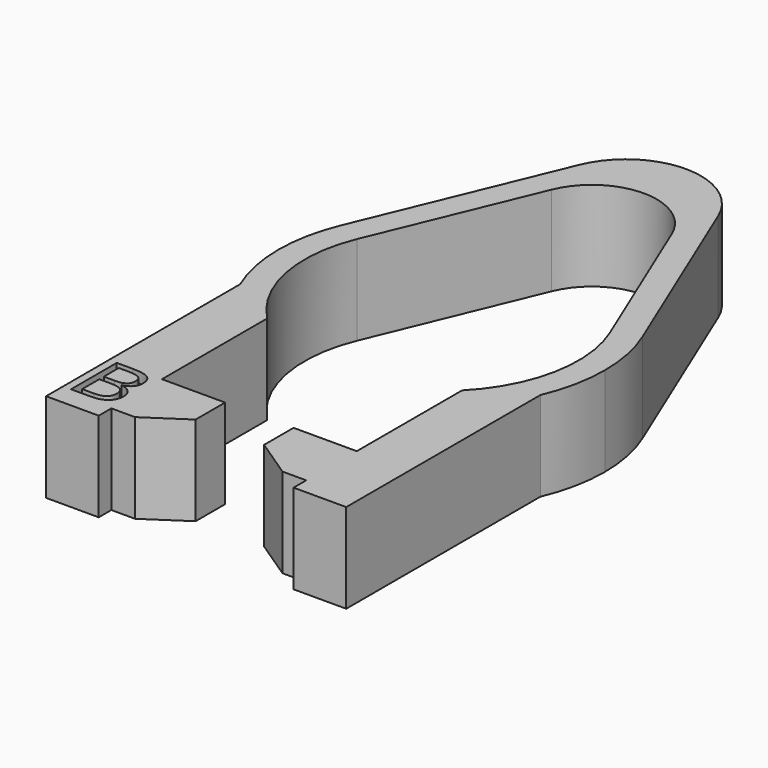
from build123d import *

# Parameters (mm, degrees)
F0_TEXT_SIZE = 7.602755999
F1_DEPTH     = 8.5
F2_DEPTH     = 1


# Not quite as in the source:
# - Text() gives the source's letters only with a copy of the font that has no kerning and outlines rounded to 1/6400 em; it was checked with that copy


with BuildPart() as f1:
    # F0 (on Top) → F1 (new body)
    with BuildSketch(Plane.XY):
        with BuildLine():
            ThreePointArc((-9.25, -9.1344129532), (-12.758649851, -2.493361983), (-12.0083127685, 4.9800024553))
            Line((-12.0083127685, 4.9800024553), (-5.6989333404, 20.1938506868))
            ThreePointArc((-5.6989333404, 20.1938506868), (0, 24), (5.6989333404, 20.1938506868))
            Line((5.6989333404, 20.1938506868), (12.0083127685, 4.9800024553))
            ThreePointArc((12.0083127685, 4.9800024553), (12.758649851, -2.493361983), (9.25, -9.1344129532))
            Line((9.25, -9.1344129532), (9.25, -12.4373429638))
            Line((9.25, -12.4373429638), (9.25, -21.6344129532))
            Line((9.25, -21.6344129532), (3.25, -21.6344129532))
            Line((3.25, -21.6344129532), (3.25, -22.6344129532))
            Line((3.25, -22.6344129532), (3.25, -25.1344129532))
            Line((3.25, -25.1344129532), (7, -27.6344129532))
            Line((7, -27.6344129532), (9.25, -27.6344129532))
            Line((9.25, -27.6344129532), (9.25, -29.1344129532))
            Line((9.25, -29.1344129532), (14.25, -29.1344129532))
            Line((14.25, -29.1344129532), (14.25, -22.6230966869))
            Line((14.25, -22.6230966869), (14.25, -6.0981554588))
            ThreePointArc((14.25, -6.0981554588), (15.1842846391, -3.1124748995), (15.5, 0))
            ThreePointArc((15.5, 0), (15.2015271786, 3.0271391507), (14.3176036855, 5.9376952352))
            Line((14.3176036855, 5.9376952352), (6.5742743873, 24.6092362465))
            ThreePointArc((6.5742743873, 24.6092362465), (0, 29), (-6.5742743873, 24.6092362465))
            Line((-6.5742743873, 24.6092362465), (-14.3176036855, 5.9376952352))
            ThreePointArc((-14.3176036855, 5.9376952352), (-15.2015271786, 3.0271391507), (-15.5, 0))
            ThreePointArc((-15.5, 0), (-15.1842846391, -3.1124748995), (-14.25, -6.0981554588))
            Line((-14.25, -6.0981554588), (-14.25, -22.6344129532))
            Line((-14.25, -22.6344129532), (-14.25, -29.1344129532))
            Line((-14.25, -29.1344129532), (-9.25, -29.1344129532))
            Line((-9.25, -29.1344129532), (-9.25, -27.6344129532))
            Line((-9.25, -27.6344129532), (-7, -27.6344129532))
            Line((-7, -27.6344129532), (-3.25, -25.1344129532))
            Line((-3.25, -25.1344129532), (-3.25, -22.6344129532))
            Line((-3.25, -22.6344129532), (-3.25, -21.6344129532))
            Line((-3.25, -21.6344129532), (-9.25, -21.6344129532))
            Line((-9.25, -21.6344129532), (-9.25, -12.4373429638))
            Line((-9.25, -12.4373429638), (-9.25, -9.1344129532))
        make_face()
        with BuildLine():
            Line((-13.5039795676, -27.1083972725), (-13.5039795676, -21.6807422476))
            Line((-13.5039795676, -21.6807422476), (-11.9703611309, -21.6807422476))
            add(Edge.make_bspline(
                [(-11.9703611309, -21.6807422476), (-10.8905321929, -21.6807422476), (-10.4076383939, -22.0038593776)],
                knots=[0, 0, 0, 1, 1, 1], degree=2))
            add(Edge.make_bspline(
                [(-10.4076383939, -22.0038593776), (-9.9247445949, -22.3269765075), (-9.9247445949, -23.0242917843)],
                knots=[0, 0, 0, 1, 1, 1], degree=2))
            add(Edge.make_bspline(
                [(-9.9247445949, -23.0242917843), (-9.9247445949, -23.5077795486), (-10.1938108814, -23.8213932336)],
                knots=[0, 0, 0, 1, 1, 1], degree=2))
            add(Edge.make_bspline(
                [(-10.1938108814, -23.8213932336), (-10.462877168, -24.1350069185), (-10.9796269898, -24.2276655073)],
                knots=[0, 0, 0, 1, 1, 1], degree=2))
            Line((-10.9796269898, -24.2276655073), (-10.9796269898, -24.2644913566))
            add(Edge.make_bspline(
                [(-10.9796269898, -24.2644913566), (-9.7429912093, -24.4759430079), (-9.7429912093, -25.5640874602)],
                knots=[0, 0, 0, 1, 1, 1], degree=2))
            add(Edge.make_bspline(
                [(-9.7429912093, -25.5640874602), (-9.7429912093, -26.2911010026), (-10.234794488, -26.6997491376)],
                knots=[0, 0, 0, 1, 1, 1], degree=2))
            add(Edge.make_bspline(
                [(-10.234794488, -26.6997491376), (-10.7265977667, -27.1083972725), (-11.6104181516, -27.1083972725)],
                knots=[0, 0, 0, 1, 1, 1], degree=2))
            Line((-11.6104181516, -27.1083972725), (-13.5039795676, -27.1083972725))
        make_face(mode=Mode.SUBTRACT)
        with Locations((-14.25, -27.1083972725)):
            Text('B', F0_TEXT_SIZE, font='Open Sans', text_align=(TextAlign.LEFT, TextAlign.BOTTOM))
        with BuildLine():
            Line((-11.7921715372, -24.538903331), (-12.8731884058, -24.538903331))
            Line((-12.8731884058, -24.538903331), (-12.8731884058, -26.5702646995))
            Line((-12.8731884058, -26.5702646995), (-11.7399025897, -26.5702646995))
            add(Edge.make_bspline(
                [(-11.7399025897, -26.5702646995), (-11.0829769541, -26.5702646995), (-10.7509503445, -26.3160475458)],
                knots=[0, 0, 0, 1, 1, 1], degree=2))
            add(Edge.make_bspline(
                [(-10.7509503445, -26.3160475458), (-10.4189237349, -26.061830392), (-10.4189237349, -25.5189460965)],
                knots=[0, 0, 0, 1, 1, 1], degree=2))
            add(Edge.make_bspline(
                [(-10.4189237349, -25.5189460965), (-10.4189237349, -25.0140755809), (-10.7586718936, -24.776489456)],
                knots=[0, 0, 0, 1, 1, 1], degree=2))
            add(Edge.make_bspline(
                [(-10.7586718936, -24.776489456), (-11.0984200523, -24.538903331), (-11.7921715372, -24.538903331)],
                knots=[0, 0, 0, 1, 1, 1], degree=2))
        make_face()
        with BuildLine():
            Line((-12.8731884058, -22.227190335), (-12.8731884058, -24.0043345498))
            Line((-12.8731884058, -24.0043345498), (-11.8337491091, -24.0043345498))
            add(Edge.make_bspline(
                [(-11.8337491091, -24.0043345498), (-11.1649441673, -24.0043345498), (-10.8715253029, -23.7946647945)],
                knots=[0, 0, 0, 1, 1, 1], degree=2))
            add(Edge.make_bspline(
                [(-10.8715253029, -23.7946647945), (-10.5781064386, -23.5849950392), (-10.5781064386, -23.088440038)],
                knots=[0, 0, 0, 1, 1, 1], degree=2))
            add(Edge.make_bspline(
                [(-10.5781064386, -23.088440038), (-10.5781064386, -22.6310867475), (-10.9047873604, -22.4291385412)],
                knots=[0, 0, 0, 1, 1, 1], degree=2))
            add(Edge.make_bspline(
                [(-10.9047873604, -22.4291385412), (-11.2314682823, -22.227190335), (-11.9442266572, -22.227190335)],
                knots=[0, 0, 0, 1, 1, 1], degree=2))
            Line((-11.9442266572, -22.227190335), (-12.8731884058, -22.227190335))
        make_face()
    extrude(amount=-F1_DEPTH)

    # F0 (on Top) → F2 (cut)
    with BuildSketch(Plane.XY):
        with Locations((-14.25, -27.1083972725)):
            Text('B', F0_TEXT_SIZE, font='Open Sans', text_align=(TextAlign.LEFT, TextAlign.BOTTOM))
    extrude(amount=-F2_DEPTH, mode=Mode.SUBTRACT)


solid = f1.part
